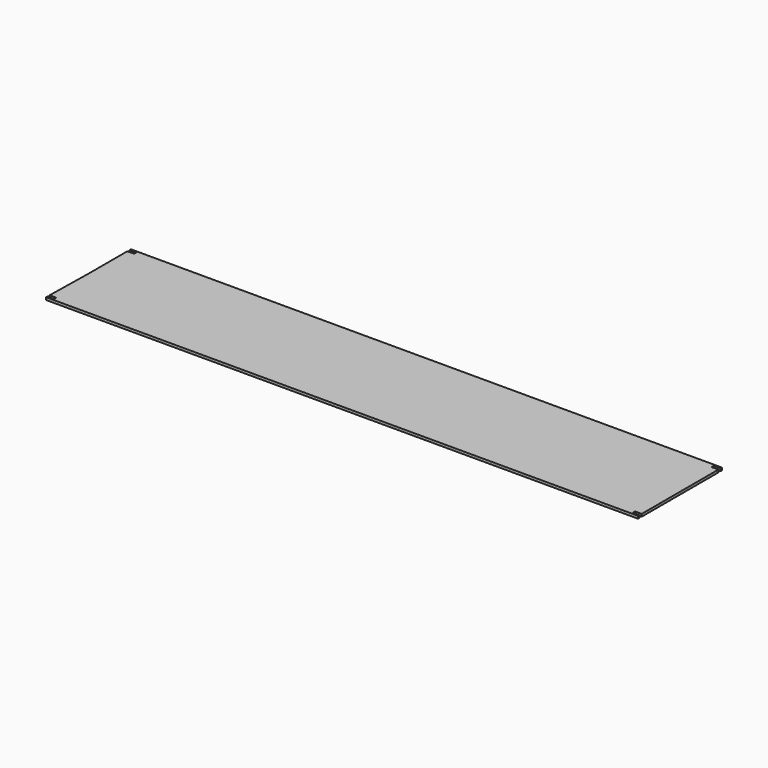
from build123d import *

# Parameters (mm, degrees)
F1_DEPTH = 0.75
F3_DEPTH = 0.75
F4_W     = 2
F4_H     = 0.8
F5_DEPTH = 25
F6_W     = 2
F6_H     = 0.8
F7_DEPTH = 0.751
F8_W     = 2
F8_H     = 0.8
F9_DEPTH = 0.751


with BuildPart() as f1:
    # F0 (on Top) → F1 (new body)
    with BuildSketch(Plane.XY):
        Polygon((-87.5160314443, 15.5), (-87.5160314443, 0), (-87.8127528557, -15.5), (87.4839685557, -15.5), (87.4839685557, 15.5), align=None)
    extrude(amount=F1_DEPTH)

    # F2 (on face) → F3 (cut, through all)
    with BuildSketch(Plane.XY.offset(0.75)):
        Polygon((-87.7885993427, -14.2382796203), (-87.8031811973, -15), (-85.8035475632, -15.0382796203), (-85.8035475632, -14.2382796203), align=None)
    extrude(amount=-F3_DEPTH, mode=Mode.SUBTRACT)

    # F4 (on face) → F5 (cut)
    with BuildSketch(Plane.XY.offset(0.75)):
        with Locations((-86.5160314443, 14.6)):
            Rectangle(F4_W, F4_H)
    extrude(amount=-F5_DEPTH, mode=Mode.SUBTRACT)

    # F6 (on face) → F7 (cut, through all)
    with BuildSketch(Plane.XY.offset(0.75)):
        with Locations((86.4839685557, 14.6)):
            Rectangle(F6_W, F6_H)
    extrude(amount=-F7_DEPTH, mode=Mode.SUBTRACT)

    # F8 (on face) → F9 (cut, through all)
    with BuildSketch(Plane.XY.offset(0.75)):
        with Locations((86.4839685557, -14.6)):
            Rectangle(F8_W, F8_H)
    extrude(amount=-F9_DEPTH, mode=Mode.SUBTRACT)


solid = f1.part
